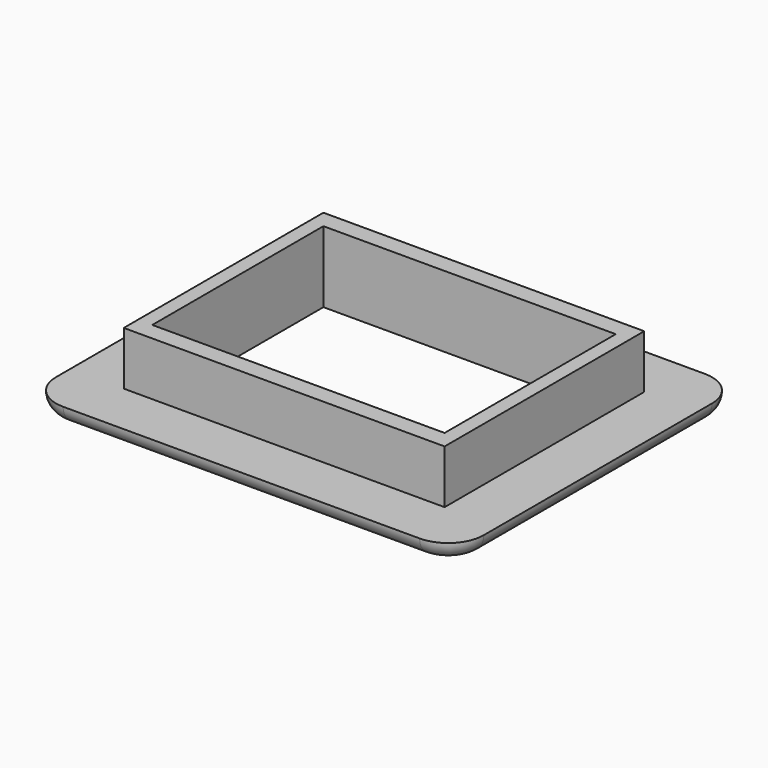
from build123d import *

# Parameters (mm, degrees)
F0_W     = 90
F0_H     = 70
F0_W_2   = 82
F0_H_2   = 60
F1_DEPTH = 5
F2_DEPTH = 20
F3_DEPTH = 20
F4_R     = 4.99999


# Not quite as in the source:
# - a fillet or chamfer is up to 0.001 mm smaller than in the source, because OpenCascade refuses the exact size
# - a feature names something its author has since deleted; it is built from what else it names


with BuildPart() as f1:
    # F0 (on Top) → F1 (new body)
    with BuildSketch(Plane.XY):
        with BuildLine():
            Line((-50, -50), (50, -50))
            ThreePointArc((50, -50), (57.0710678119, -47.0710678119), (60, -40))
            Line((60, -40), (60, 40))
            ThreePointArc((60, 40), (57.0710678119, 47.0710678119), (50, 50))
            Line((50, 50), (-50, 50))
            ThreePointArc((-50, 50), (-57.0710678119, 47.0710678119), (-60, 40))
            Line((-60, 40), (-60, -40))
            ThreePointArc((-60, -40), (-57.0710678119, -47.0710678119), (-50, -50))
        make_face()
        Rectangle(F0_W, F0_H, mode=Mode.SUBTRACT)
        Rectangle(F0_W, F0_H)
        Rectangle(F0_W_2, F0_H_2, mode=Mode.SUBTRACT)
    extrude(amount=F1_DEPTH)

    # F0 (on Top) → F2 (join)
    with BuildSketch(Plane.XY):
        Rectangle(F0_W, F0_H)
        Rectangle(F0_W_2, F0_H_2, mode=Mode.SUBTRACT)
        Rectangle(F0_W_2, F0_H_2)
    extrude(amount=F2_DEPTH)

    # F0 (on Top) → F3 (cut)
    with BuildSketch(Plane.XY):
        Rectangle(F0_W_2, F0_H_2)
    extrude(amount=F3_DEPTH, mode=Mode.SUBTRACT)

    # F4 (radius 5 in the source; OpenCascade refuses exactly that, so slightly less here)
    f4_edges = [f1.edges().sort_by_distance(p)[0] for p in [
        (57.071068, -47.071068, 0),
    ]]
    fillet(f4_edges, radius=F4_R)


solid = f1.part
